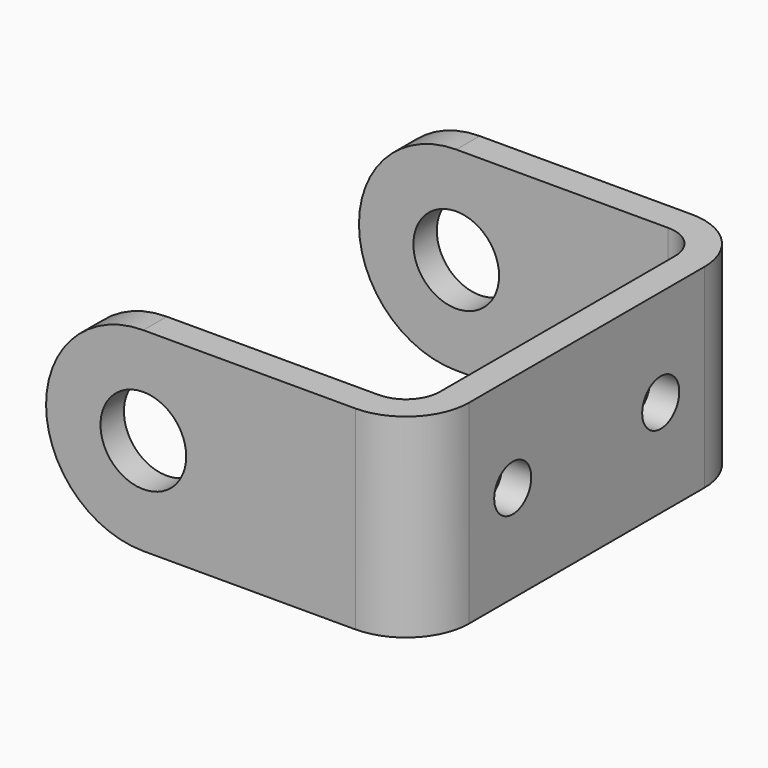
from build123d import *

# Parameters (mm, degrees)
F1_DEPTH = 11.34999
F2_R     = 5.674985
F3_R     = 2.5
F4_DEPTH = 24.53132
F5_R     = 3.69316
F6_R     = 1.98374
F7_R     = 1.35255
F8_DEPTH = 1.70942


# Not quite as in the source:
# - a fillet or chamfer is up to 0.001 mm smaller than in the source, because OpenCascade refuses the exact size


with BuildPart() as f1:
    # F0 (on Top) → F1 (new body)
    with BuildSketch(Plane.XY):
        Polygon((-20.0249917, 0), (0, 0), (0, -21.11248), (-20.0249917, -21.11248), (-20.0249917, -22.8219), (1.70942, -22.8219), (1.70942, 1.70942), (-20.0249917, 1.70942), align=None)
    extrude(amount=F1_DEPTH)

    # F2 (radius 5.674995 in the source; OpenCascade refuses exactly that, so slightly less here)
    f2_edges = [f1.edges().sort_by_distance(p)[0] for p in [
        (-20.024992, -21.96719, 11.34999),
        (-20.024992, -21.96719, 0),
        (-20.024992, 0.85471, 11.34999),
        (-20.024992, 0.85471, 0),
    ]]
    fillet(f2_edges, radius=F2_R)

    # F3 (on face) → F4 (cut, through all)
    with BuildSketch(Plane.XZ.offset(22.8219)):
        with Locations((-14.3499967, 5.674995)):
            Circle(F3_R)
    extrude(amount=-F4_DEPTH, mode=Mode.SUBTRACT)

    # F5
    f5_edges = [f1.edges().sort_by_distance(p)[0] for p in [
        (1.70942, -22.8219, 5.674995),
        (1.70942, 1.70942, 5.674995),
    ]]
    fillet(f5_edges, radius=F5_R)

    # F6
    f6_edges = [f1.edges().sort_by_distance(p)[0] for p in [
        (0, -21.11248, 5.674995),
        (0, 0, 5.674995),
    ]]
    fillet(f6_edges, radius=F6_R)

    # F7 (on face) → F8 (cut, through all)
    with BuildSketch(Plane(origin=(0, 0, 0), x_dir=(0, -1, 0), z_dir=(-1, 0, 0))):
        with Locations((15.95374, 5.674995)):
            Circle(F7_R)
        with Locations((5.15874, 5.674995)):
            Circle(F7_R)
    extrude(amount=-F8_DEPTH, mode=Mode.SUBTRACT)


solid = f1.part
